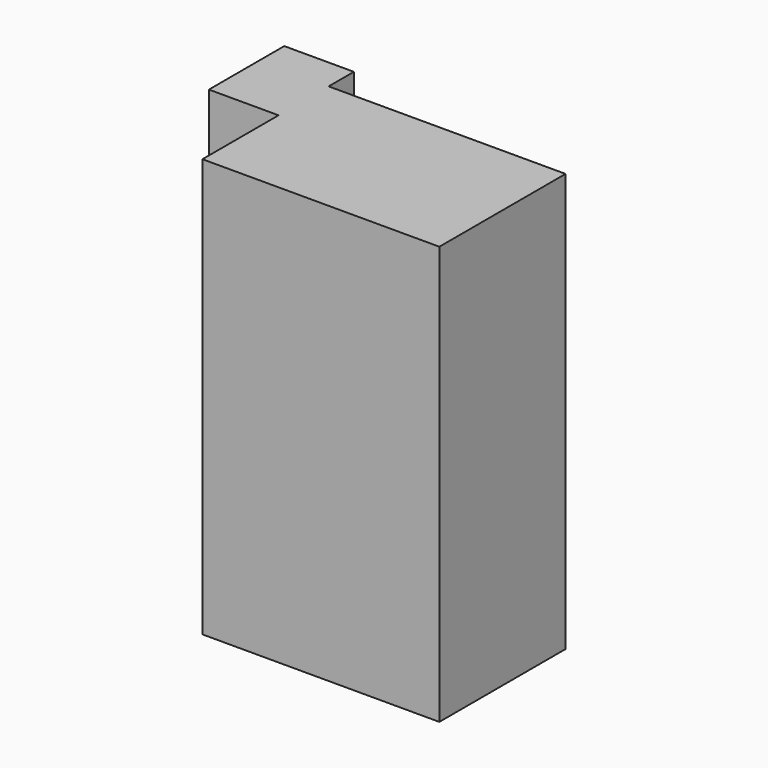
from build123d import *

# Parameters (mm, degrees)
F3_DEPTH = 152.4


# Not quite as in the source:
# - a feature of the source that left no trace in its solid (it failed there, or was rolled back) is left out


with BuildPart() as f3:
    # F2 (on Top) → F3 (new body)
    with BuildSketch(Plane.XY):
        Polygon((-35.4751944542, 0), (-35.4751944542, -34.6453338861), (50.8269667625, -34.6453338861), (50.8269667625, 22.8202939034), (-35.4751944542, 22.8202939034), align=None)
        Polygon((-60.8430989087, 0), (-35.4751944542, 0), (-35.4751944542, 22.8202939034), (-35.4751944542, 34.3115627766), (-60.8430989087, 34.3115627766), align=None)
    extrude(amount=-F3_DEPTH)


solid = f3.part
